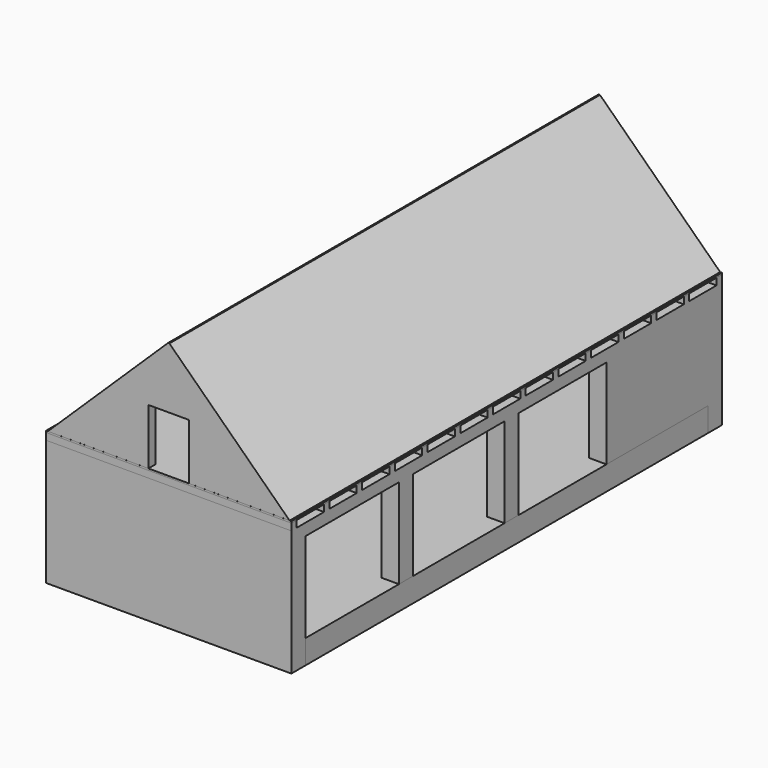
from build123d import *

# Parameters (mm, degrees)
F0_W      = 520
F0_H      = 3240
F0_H_2    = 520
F0_H_3    = 3380
F0_H_4    = 3450
F1_DEPTH  = 10
F2_DEPTH  = 3350
F3_W      = 520
F3_H      = 11110
F4_DEPTH  = 350
F5_W      = 7240
F5_H      = 200
F6_DEPTH  = 200
F7_W      = 7240
F7_H      = 15890
F8_DEPTH  = 3500
F9_SIZE2  = 3499.99999
F9_SIZE   = 3599.99999
F10_T     = 260
F11_W     = 1200
F11_H     = 1700
F12_DEPTH = 260
F13_W     = 6720
F13_H     = 14850
F14_DEPTH = 700
F15_W     = 7240
F15_H     = 15891
F16_DEPTH = 50


# Not quite as in the source:
# - a fillet or chamfer is up to 0.001 mm smaller than in the source, because OpenCascade refuses the exact size
# - a shell that OpenCascade refuses in one call is made with other operations: the cavity is built on its own and cut out


with BuildPart() as f1:
    # F0 (on Top) → F1 (new body)
    with BuildSketch(Plane.XY):
        Polygon((-3374.345998764, -8413.8299859681), (-3374.345998764, 6436.1700140319), (2825.654001236, 6436.1700140319), (2825.654001236, 2696.170014032), (3345.654001236, 2696.170014032), (3345.654001236, 6956.1700140319), (-3894.345998764, 6956.1700140319), (-3894.345998764, -8933.8299859681), (3345.654001236, -8933.8299859681), (3345.654001236, -8413.8299859681), (2825.654001236, -8413.8299859681), align=None)
        Polygon((2825.654001236, 6436.1700140319), (-3374.345998764, 6436.1700140319), (-3374.345998764, -8413.8299859681), (2825.654001236, -8413.8299859681), (2825.654001236, -4963.8299859681), (2825.654001236, -4443.829985968), (2825.654001236, -1063.8299859681), (2825.654001236, -543.829985968), (2825.654001236, 2696.170014032), align=None)
        with Locations((3085.654001236, 1076.170014032)):
            Rectangle(F0_W, F0_H)
        with Locations((3085.654001236, -803.829985968)):
            Rectangle(F0_W, F0_H_2)
        with Locations((3085.654001236, -2753.829985968)):
            Rectangle(F0_W, F0_H_3)
        with Locations((3085.654001236, -6688.8299859681)):
            Rectangle(F0_W, F0_H_4)
        with Locations((3085.654001236, -4703.8299859681)):
            Rectangle(F0_W, F0_H_2)
    extrude(amount=-F1_DEPTH)

    # F0 (on Top) → F2 (join)
    with BuildSketch(Plane.XY):
        with Locations((3085.654001236, -803.829985968)):
            Rectangle(F0_W, F0_H_2)
        with Locations((3085.654001236, -4703.8299859681)):
            Rectangle(F0_W, F0_H_2)
        Polygon((-3374.345998764, -8413.8299859681), (-3374.345998764, 6436.1700140319), (2825.654001236, 6436.1700140319), (2825.654001236, 2696.170014032), (3345.654001236, 2696.170014032), (3345.654001236, 6956.1700140319), (-3894.345998764, 6956.1700140319), (-3894.345998764, -8933.8299859681), (3345.654001236, -8933.8299859681), (3345.654001236, -8413.8299859681), (2825.654001236, -8413.8299859681), align=None)
    extrude(amount=F2_DEPTH)

    # F3 (on face) → F4 (join)
    with BuildSketch(Plane.XY.offset(3350)):
        Polygon((3345.654001236, 6956.1700140319), (-3894.345998764, 6956.1700140319), (-3894.345998764, -8933.8299859681), (3345.654001236, -8933.8299859681), (3345.654001236, -8413.8299859681), (2825.654001236, -8413.8299859681), (-3374.345998764, -8413.8299859681), (-3374.345998764, 6436.1700140319), (2825.654001236, 6436.1700140319), (2825.654001236, 2696.170014032), (3345.654001236, 2696.170014032), align=None)
        with Locations((3085.654001236, -2858.8299859681)):
            Rectangle(F3_W, F3_H)
    extrude(amount=F4_DEPTH)

    # F5 (on face) → F6 (join)
    with BuildSketch(Plane.XY.offset(3700)):
        with Locations((-274.345998764, 6856.1700140319)):
            Rectangle(F5_W, F5_H)
        with Locations((-274.345998764, 5649.1700140319)):
            Rectangle(F5_W, F5_H)
        with Locations((-274.345998764, 4442.1700140319)):
            Rectangle(F5_W, F5_H)
        with Locations((-274.345998764, 3235.1700140319)):
            Rectangle(F5_W, F5_H)
        with Locations((-274.345998764, 2028.1700140319)):
            Rectangle(F5_W, F5_H)
        with Locations((-274.345998764, 821.1700140319)):
            Rectangle(F5_W, F5_H)
        with Locations((-274.345998764, -385.8299859681)):
            Rectangle(F5_W, F5_H)
        with Locations((-274.345998764, -1592.8299859681)):
            Rectangle(F5_W, F5_H)
        with Locations((-274.345998764, -2799.8299859681)):
            Rectangle(F5_W, F5_H)
        with Locations((-274.345998764, -4006.8299859681)):
            Rectangle(F5_W, F5_H)
        with Locations((-274.345998764, -5213.8299859681)):
            Rectangle(F5_W, F5_H)
        with Locations((-274.345998764, -6420.8299859681)):
            Rectangle(F5_W, F5_H)
        with Locations((-274.345998764, -7627.8299859681)):
            Rectangle(F5_W, F5_H)
        with Locations((-274.345998764, -8834.8299859681)):
            Rectangle(F5_W, F5_H)
    extrude(amount=F6_DEPTH)


with BuildPart() as f8:
    # F7 (on face) → F8 (new body)
    with BuildSketch(Plane.XY.offset(3900)):
        with Locations((-274.345998764, -988.8299859681)):
            Rectangle(F7_W, F7_H)
    extrude(amount=F8_DEPTH)

    # F9 (size 3600 and 3500 in the source; OpenCascade refuses exactly that, so slightly less here)
    f9_edges = [f8.edges().sort_by_distance(p)[0] for p in [
        (-3894.345999, -988.829986, 7400),
        (3345.654001, -988.829986, 7400),
    ]]
    f9_side = f8.faces().sort_by_distance((-274.345999, -988.829986, 7400))[0]
    chamfer(f9_edges, length=F9_SIZE, length2=F9_SIZE2, reference=f9_side)

    # F10: shell of thickness 260, made by hand


with BuildPart() as f10_core1:
    # F10_t2: copy of F8
    add(f8.part)

    # the walls: a layer under each face that stays
    f10_faces = [f10_core1.faces().sort_by_distance(p)[0] for p in [
        (-274.3459987642, -8933.8299859681, 5650.0000000001),
        (-3894.345998764, -988.8299859681, 3900.0000050002),
        (-2094.3460037642, -988.8299859681, 5650.0000050002),
        (-274.345998764, -988.8299859681, 7400),
        (3345.654001236, -988.8299859681, 3900.0000050002),
        (1545.6540062361, -988.8299859681, 5650.0000050002),
        (-274.3459987639, 6956.1700140319, 5650.0000000001),
    ]]
    thicken(f10_faces, amount=-F10_T, mode=Mode.SUBTRACT)


with BuildPart() as f8_1:
    add(f8.part)

    # what is left inside the walls is the cavity
    f10_cavity = [f10_core1.part.solids().sort_by_distance(p)[0] for p in [
        (-274.345999, -3550.496653, 3902.6),
    ]]
    add(f10_cavity, mode=Mode.SUBTRACT)

    # F11 (on face) → F12 (cut)
    with BuildSketch(Plane.XZ.offset(8933.8299859681)):
        with Locations((-274.345998764, 4750)):
            Rectangle(F11_W, F11_H)
    extrude(amount=-F12_DEPTH, mode=Mode.SUBTRACT)


with BuildPart() as f14:
    # F13 (on face) → F14 (new body)
    with BuildSketch(Plane.XY):
        with Locations((-14.345998764, -988.8299859681)):
            Rectangle(F13_W, F13_H)
    extrude(amount=F14_DEPTH)


with BuildPart() as f16:
    # F15 (on face) → F16 (new body)
    with BuildSketch(Plane.XY.offset(3900)):
        with Locations((-274.345998764, -989.3299859681)):
            Rectangle(F15_W, F15_H)
    extrude(amount=F16_DEPTH)


solid = Compound([f1.part, f8_1.part, f14.part, f16.part])
